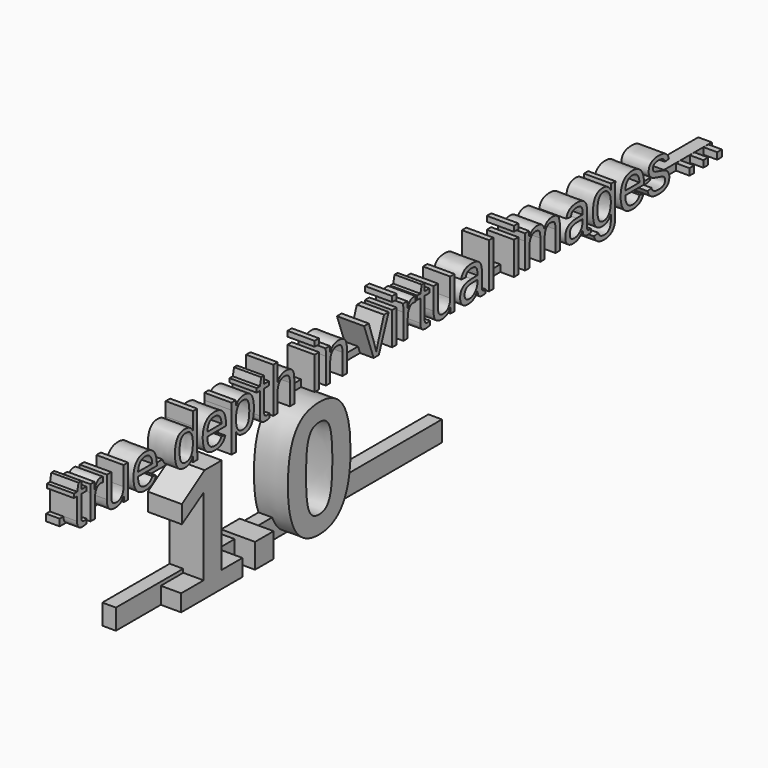
from build123d import *

# Parameters (mm, degrees)
F1_W         = 60
F1_H         = 0.5
F2_DEPTH     = 1
F0_TEXT_SIZE = 4.5819561612
F3_DEPTH     = 2
F5_W         = 30
F5_H         = 1.5
F6_DEPTH     = 1
F4_TEXT_SIZE = 12.1166224915
F7_DEPTH     = 2.5


# Not quite as in the source:
# - Text() gives the source's letters only with a copy of the font that has no kerning and outlines rounded to 1/6400 em; it was checked with that copy


with BuildPart() as f2:
    # F1 (on Right) → F2 (new body)
    with BuildSketch(Plane.YZ):
        with Locations((21.1383859832, 6.7239139581)):
            Rectangle(F1_W, F1_H)
    extrude(amount=F2_DEPTH)

    # F0 (on Right) → F3 (join)
    with BuildSketch(Plane.YZ):
        with Locations((-8.8616140168, 6.4739139581)):
            Text('true depth in virtual images ...', F0_TEXT_SIZE, font='Arimo', text_align=(TextAlign.LEFT, TextAlign.BOTTOM))
    extrude(amount=F3_DEPTH)


with BuildPart() as f6:
    # F5 (on Right) → F6 (new body)
    with BuildSketch(Plane.YZ):
        with Locations((11.3131188363, -1.6407375371)):
            Rectangle(F5_W, F5_H)
    extrude(amount=F6_DEPTH)

    # F4 (on Right) → F7 (join)
    with BuildSketch(Plane.YZ):
        with Locations((-0.3207319778, -2.3907375371)):
            Text('1.0', F4_TEXT_SIZE, font='Arimo', font_style=FontStyle.BOLD, text_align=(TextAlign.LEFT, TextAlign.BOTTOM))
    extrude(amount=F7_DEPTH)


solid = Compound([f2.part, f6.part])
